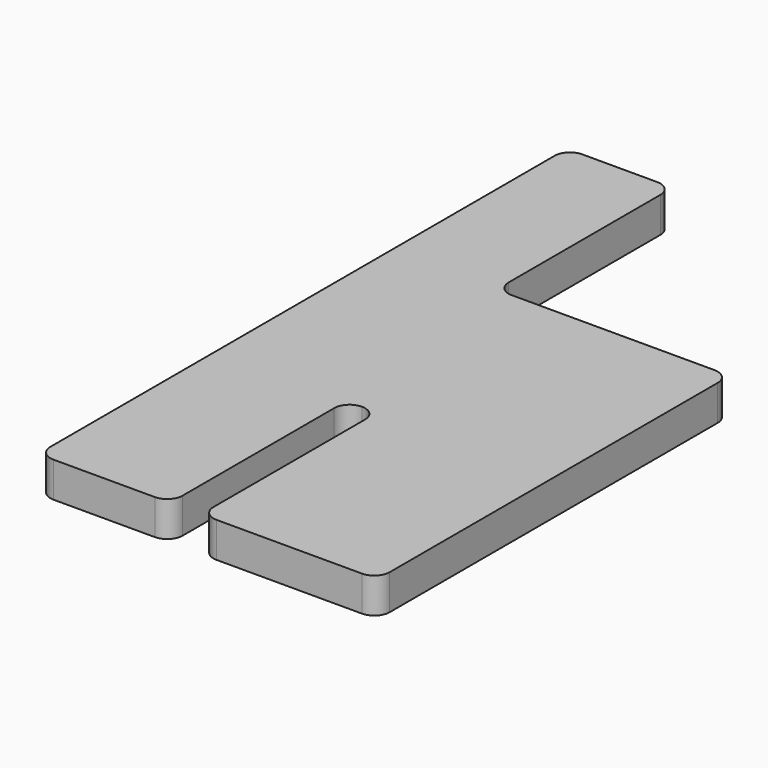
from build123d import *

# Parameters (mm, degrees)
F1_DEPTH = 2.032
F2_R     = 0.88899


# Not quite as in the source:
# - a fillet or chamfer is up to 0.001 mm smaller than in the source, because OpenCascade refuses the exact size


with BuildPart() as f1:
    # F0 (on Top) → F1 (new body)
    with BuildSketch(Plane.XY):
        Polygon((-1.524, 19.05), (-7.62, 19.05), (-7.62, -19.05), (0, -19.05), (0, -6.35), (1.778, -6.35), (1.778, -19.05), (11.938, -19.05), (11.938, 6.35), (-1.524, 6.35), align=None)
    extrude(amount=F1_DEPTH)

    # F2 (radius 0.889 in the source; OpenCascade refuses exactly that, so slightly less here)
    f2_edges = [f1.edges().sort_by_distance(p)[0] for p in [
        (-7.62, -19.05, 1.016),
        (0, -19.05, 1.016),
        (0, -6.35, 1.016),
        (1.778, -19.05, 1.016),
        (11.938, -19.05, 1.016),
        (11.938, 6.35, 1.016),
        (-1.524, 19.05, 1.016),
        (1.778, -6.35, 1.016),
        (-7.62, 19.05, 1.016),
        (-1.524, 6.35, 1.016),
    ]]
    fillet(f2_edges, radius=F2_R)


solid = f1.part
